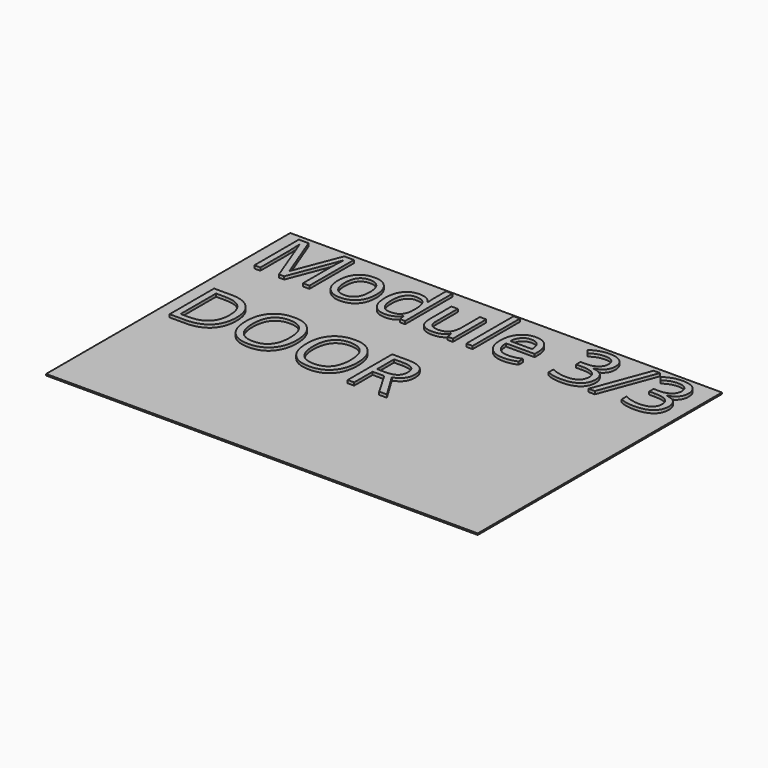
from build123d import *

# Parameters (mm, degrees)
F0_W         = 297
F0_H         = 210
F1_DEPTH     = 1
F2_TEXT_SIZE = 53.5855380197
F3_DEPTH     = 2


# Not quite as in the source:
# - Text() gives the source's letters only with a copy of the font that has no kerning and outlines rounded to 1/6400 em; it was checked with that copy


with BuildPart() as f1:
    # F0 (on Top) → F1 (new body)
    with BuildSketch(Plane.XY):
        with Locations((-47.4010080695, 34.3840229511)):
            Rectangle(F0_W, F0_H)
    extrude(amount=F1_DEPTH)

    # F2 (on face) → F3 (join)
    with BuildSketch(Plane.XY.offset(1)):
        with Locations((-190.3507038951, 94.9954763055)):
            Text('Module 3/3', F2_TEXT_SIZE, font='Open Sans', text_align=(TextAlign.LEFT, TextAlign.BOTTOM))
        with Locations((-190.3507038951, 22.1191445986)):
            Text('DOOR', F2_TEXT_SIZE, font='Open Sans', text_align=(TextAlign.LEFT, TextAlign.BOTTOM))
    extrude(amount=F3_DEPTH)


solid = f1.part
